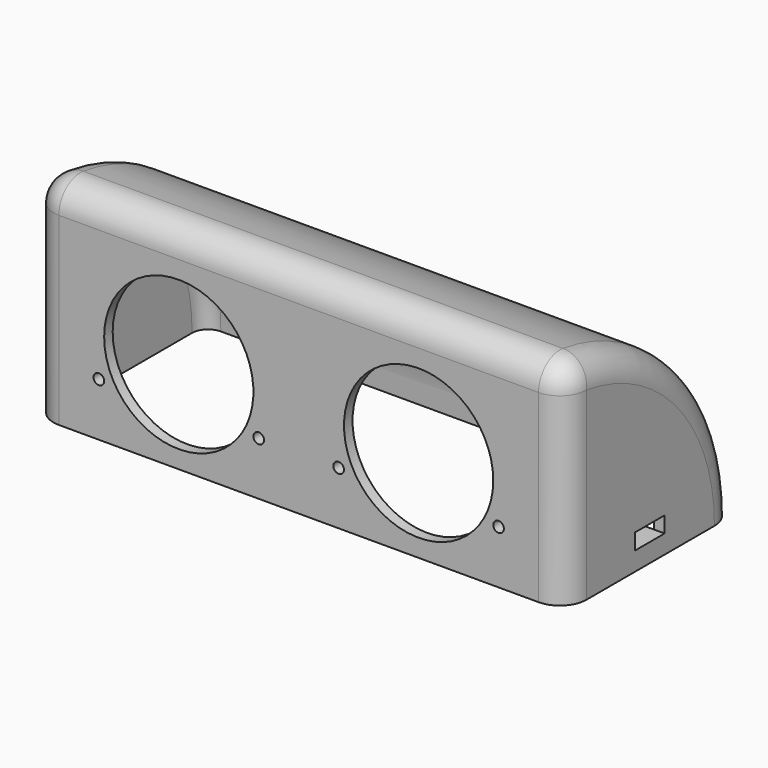
from build123d import *

# Parameters (mm, degrees)
F1_DEPTH  = 50
F2_R      = 5
F3_T      = -2
F4_R      = 14
F4_R_2    = 1
F5_DEPTH  = 2
F8_R      = 1
F9_DEPTH  = 10
F10_W     = 7
F10_H     = 3
F11_DEPTH = 2
F12_W     = 7
F12_H     = 3.5
F13_DEPTH = 8


with BuildPart() as f1:
    # F0 (on Right) → F1 (new body)
    with BuildSketch(Plane.YZ):
        with BuildLine():
            Line((-23.8863006731, 0), (16.1136993269, 0))
            ThreePointArc((16.1136993269, 0), (4.3979705744, 28.2842712475), (-23.8863006731, 40))
            Line((-23.8863006731, 40), (-23.8863006731, 0))
        make_face()
    extrude(amount=F1_DEPTH)

    # F2
    f2_edges = [f1.edges().sort_by_distance(p)[0] for p in [
        (25, -23.886301, 40),
        (50, 4.397971, 28.284271),
        (50, -23.886301, 20),
    ]]
    fillet(f2_edges, radius=F2_R)

    # F3
    f3_openings = [f1.faces().sort_by_distance(p)[0] for p in [
        (0, -6.826337, 16.860621),
        (24.871175, -3.886301, 0),
    ]]
    offset(amount=F3_T, openings=f3_openings)

    # F4 (on face) → F5 (cut, through all)
    with BuildSketch(Plane.XZ.offset(23.8863006731)):
        with Locations((22.5, 17.3205080757)):
            Circle(F4_R)
        with Locations((7.5, 10)):
            Circle(F4_R_2)
        with Locations((37.5, 10)):
            Circle(F4_R_2)
    extrude(amount=-F5_DEPTH, mode=Mode.SUBTRACT)

    # F6: F1 across plane


with BuildPart() as f1_1:
    add(f1.part)
    add(f1.part.mirror(Plane.YZ))

    # F8 (on face) → F9 (cut)
    with BuildSketch(Plane.XZ.offset(-16.1136993269)):
        with Locations((0, 5)):
            Circle(F8_R)
    extrude(amount=F9_DEPTH, mode=Mode.SUBTRACT)

    # F10 (on face) → F11 (cut, through all)
    with BuildSketch(Plane.YZ.offset(50)):
        with Locations((-4.0657925974, 5)):
            Rectangle(F10_W, F10_H)
    extrude(amount=-F11_DEPTH, mode=Mode.SUBTRACT)

    # F12 (on face) → F13 (join)
    with BuildSketch(Plane(origin=(48, 0, 0), x_dir=(0, -1, 0), z_dir=(-1, 0, 0))):
        with Locations((4.0657925974, 1.75)):
            Rectangle(F12_W, F12_H)
    extrude(amount=F13_DEPTH)


solid = f1_1.part
